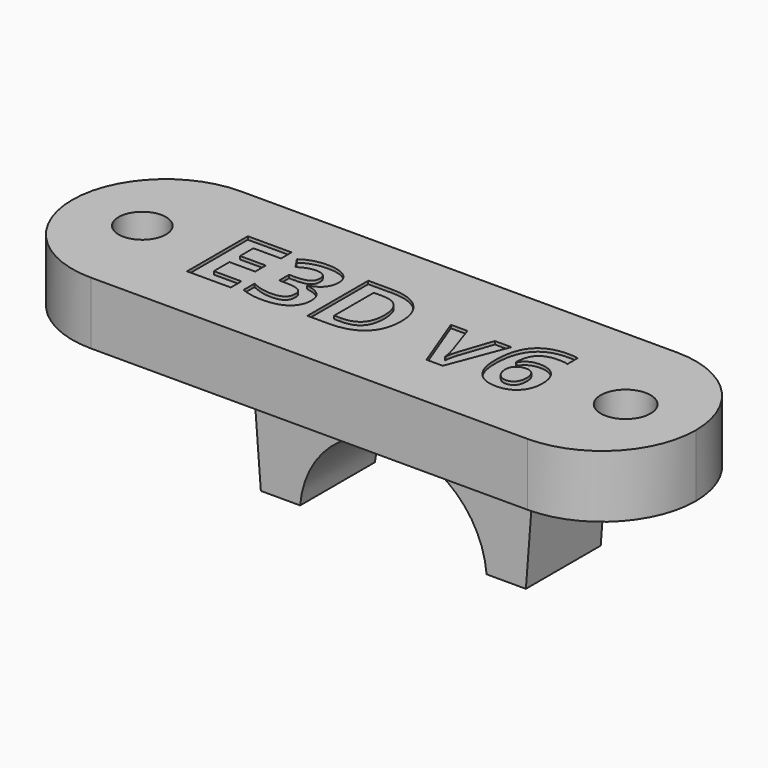
from build123d import *

# Parameters (mm, degrees)
F0_W         = 40
F0_H         = 12
F0_R         = 1.5202045648
F0_R_2       = 1.6
F1_DEPTH     = 4
F3_DEPTH     = 3
F4_R         = 5.99999
F5_TEXT_SIZE = 6.8289367047
F6_DEPTH     = 0.2


# Not quite as in the source:
# - a fillet or chamfer is up to 0.001 mm smaller than in the source, because OpenCascade refuses the exact size
# - Text() gives the source's letters only with a copy of the font that has no kerning and outlines rounded to 1/6400 em; it was checked with that copy


with BuildPart() as f1:
    # F0 (on Top) → F1 (new body)
    with BuildSketch(Plane.XY):
        Rectangle(F0_W, F0_H)
        with Locations((-15.5, 0)):
            Circle(F0_R, mode=Mode.SUBTRACT)
        with Locations((15.5, 0)):
            Circle(F0_R_2, mode=Mode.SUBTRACT)
    extrude(amount=F1_DEPTH)

    # F2 (on Front) → F3 (join, symmetric)
    with BuildSketch(Plane.XZ):
        with BuildLine():
            Line((-6, 0), (-5.5, -6.5))
            Line((-5.5, -6.5), (-2.9791303716, -6.5))
            ThreePointArc((-2.9791303716, -6.5), (3, -1), (8.9791303716, -6.5))
            Line((8.9791303716, -6.5), (11.5, -6.5))
            Line((11.5, -6.5), (12, 0))
            Line((12, 0), (-6, 0))
        make_face()
    extrude(amount=F3_DEPTH, both=True)

    # F4 (radius 6 in the source; OpenCascade refuses exactly that, so slightly less here)
    f4_edges = [f1.edges().sort_by_distance(p)[0] for p in [
        (20, 6, 2),
        (20, -6, 2),
        (-20, -6, 2),
        (-20, 6, 2),
    ]]
    fillet(f4_edges, radius=F4_R)

    # F5 (on face) → F6 (cut)
    with BuildSketch(Plane.XY.offset(4)):
        with Locations((-11.2805498191, -2.4584172137)):
            Text('E3D v6', F5_TEXT_SIZE, font='Open Sans', font_style=FontStyle.BOLD, text_align=(TextAlign.LEFT, TextAlign.BOTTOM))
    extrude(amount=-F6_DEPTH, mode=Mode.SUBTRACT)


solid = f1.part
